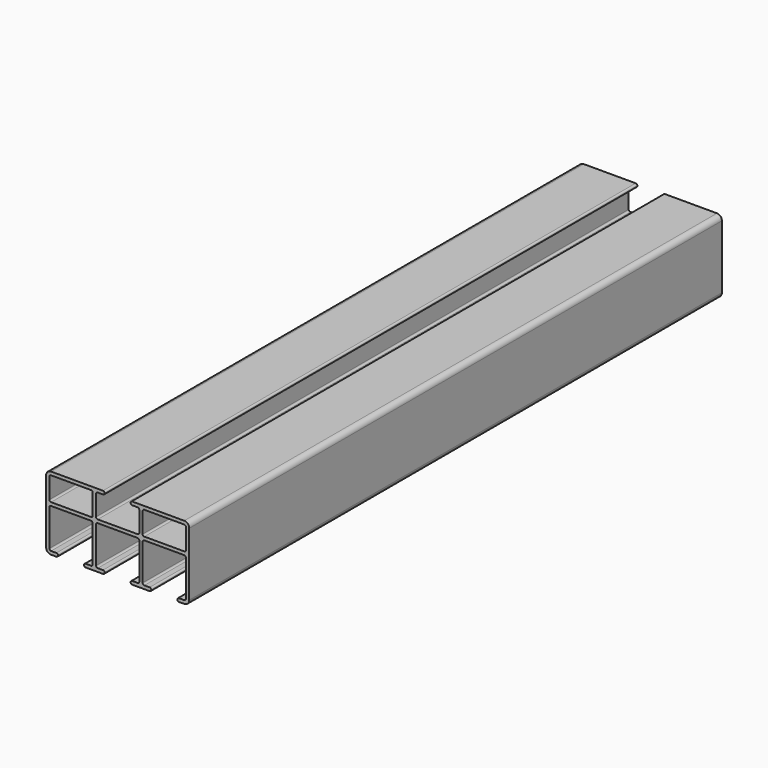
from build123d import *

# Parameters (mm, degrees)
F1_DEPTH = 200


# Not quite as in the source:
# - a pattern or mirror of a feature is missing from the dataset's text; its kind, count and spacing are read off the source's solid


with BuildPart() as f1:
    # F0 (on Front) → F1 (new body)
    with BuildSketch(Plane.XZ):
        with BuildLine():
            ThreePointArc((-3.9, 21.5), (-4.0464466094, 21.8535533906), (-4.4, 22))
            Line((-4.4, 22), (-20, 22))
            ThreePointArc((-20, 22), (-21.0606601718, 21.5606601718), (-21.5, 20.5))
            Line((-21.5, 20.5), (-21.5, 1.5))
            ThreePointArc((-21.5, 1.5), (-21.0606601718, 0.4393398282), (-20, 0))
            Line((-20, 0), (-18.4, 0))
            ThreePointArc((-18.4, 0), (-18.0464466094, 0.1464466094), (-17.9, 0.5))
            ThreePointArc((-17.9, 0.5), (-18.0464466094, 0.8535533906), (-18.4, 1))
            Line((-18.4, 1), (-20, 1))
            ThreePointArc((-20, 1), (-20.3535533906, 1.1464466094), (-20.5, 1.5))
            Line((-20.5, 1.5), (-20.5, 12.4))
            ThreePointArc((-20.5, 12.4), (-20.3535533906, 12.7535533906), (-20, 12.9))
            Line((-20, 12.9), (-8, 12.9))
            ThreePointArc((-8, 12.9), (-7.6464466094, 12.7535533906), (-7.5, 12.4))
            Line((-7.5, 12.4), (-7.5, 1.5))
            ThreePointArc((-7.5, 1.5), (-7.6464466094, 1.1464466094), (-8, 1))
            Line((-8, 1), (-9.6, 1))
            ThreePointArc((-9.6, 1), (-9.9535533906, 0.8535533906), (-10.1, 0.5))
            ThreePointArc((-10.1, 0.5), (-9.9535533906, 0.1464466094), (-9.6, 0))
            Line((-9.6, 0), (-4.4, 0))
            ThreePointArc((-4.4, 0), (-4.0464466094, 0.1464466094), (-3.9, 0.5))
            ThreePointArc((-3.9, 0.5), (-4.0464466094, 0.8535533906), (-4.4, 1))
            Line((-4.4, 1), (-6, 1))
            ThreePointArc((-6, 1), (-6.3535533906, 1.1464466094), (-6.5, 1.5))
            Line((-6.5, 1.5), (-6.5, 12.4))
            ThreePointArc((-6.5, 12.4), (-6.3535533906, 12.7535533906), (-6, 12.9))
            Line((-6, 12.9), (0, 12.9))
            Line((0, 12.9), (0, 13.9))
            Line((0, 13.9), (-6, 13.9))
            ThreePointArc((-6, 13.9), (-6.3535533906, 14.0464466094), (-6.5, 14.4))
            Line((-6.5, 14.4), (-6.5, 20.5))
            ThreePointArc((-6.5, 20.5), (-6.3535533906, 20.8535533906), (-6, 21))
            Line((-6, 21), (-4.4, 21))
            ThreePointArc((-4.4, 21), (-4.0464466094, 21.1464466094), (-3.9, 21.5))
        make_face()
        with BuildLine():
            Line((-8, 13.9), (-20, 13.9))
            ThreePointArc((-20, 13.9), (-20.3535533906, 14.0464466094), (-20.5, 14.4))
            Line((-20.5, 14.4), (-20.5, 20.5))
            ThreePointArc((-20.5, 20.5), (-20.3535533906, 20.8535533906), (-20, 21))
            Line((-20, 21), (-8, 21))
            ThreePointArc((-8, 21), (-7.6464466094, 20.8535533906), (-7.5, 20.5))
            Line((-7.5, 20.5), (-7.5, 14.4))
            ThreePointArc((-7.5, 14.4), (-7.6464466094, 14.0464466094), (-8, 13.9))
        make_face(mode=Mode.SUBTRACT)
    extrude(amount=-F1_DEPTH)

    # F1_copies: F1 across plane


with BuildPart() as f1_1:
    add(f1.part)
    add(f1.part.mirror(Plane(origin=(0, 0, 0), x_dir=(0, 0, 1), z_dir=(1, 0, 0))))


solid = f1_1.part
